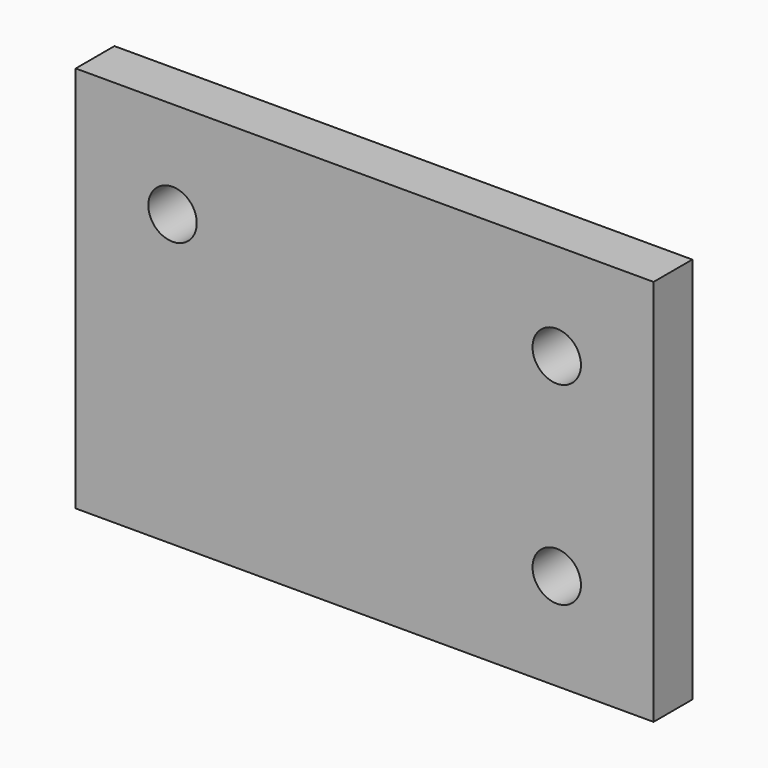
from build123d import *

# Parameters (mm, degrees)
F0_R     = 5
F1_DEPTH = 10


# Not quite as in the source:
# - the program builds the solid bodies; features that only make, move or delete a surface that nothing else refers to are left out


with BuildPart() as f1:
    # F0 (on Front) → F1 (new body)
    with BuildSketch(Plane.XZ):
        Polygon((45.889818927, 55.3569364734), (-73.4539608263, 55.3569364734), (-73.4539608263, 35.3569364734), (-73.4539608263, 5.3569364734), (45.889818927, 5.3569364734), (45.889818927, 35.3569364734), align=None)
        with BuildLine():
            ThreePointArc((-48.4539608263, 35.3569364734), (-53.4539608263, 30.3569364734), (-58.4539608263, 35.3569364734))
            ThreePointArc((-58.4539608263, 35.3569364734), (-53.4539608263, 40.3569364734), (-48.4539608263, 35.3569364734))
        make_face(mode=Mode.SUBTRACT)
        with Locations((25.889818927, 35.3569364734)):
            Circle(F0_R, mode=Mode.SUBTRACT)
        with BuildLine():
            Line((45.889818927, 5.3569364734), (-73.4539608263, 5.3569364734))
            Line((-73.4539608263, 5.3569364734), (-73.4539608263, -4.6430635266))
            Line((-73.4539608263, -4.6430635266), (20.889818927, -4.6430635266))
            ThreePointArc((20.889818927, -4.6430635266), (25.889818927, 0.3569364734), (30.889818927, -4.6430635266))
            Line((30.889818927, -4.6430635266), (45.889818927, -4.6430635266))
            Line((45.889818927, -4.6430635266), (45.889818927, 5.3569364734))
        make_face()
        with BuildLine():
            Line((20.889818927, -4.6430635266), (-73.4539608263, -4.6430635266))
            Line((-73.4539608263, -4.6430635266), (-73.4539608263, -24.6430635266))
            Line((-73.4539608263, -24.6430635266), (25.4732109606, -24.6430635266))
            Line((25.4732109606, -24.6430635266), (45.889818927, -24.6430635266))
            Line((45.889818927, -24.6430635266), (45.889818927, -4.6430635266))
            Line((45.889818927, -4.6430635266), (30.889818927, -4.6430635266))
            ThreePointArc((30.889818927, -4.6430635266), (25.889818927, -9.6430635266), (20.889818927, -4.6430635266))
        make_face()
    extrude(amount=F1_DEPTH)


solid = f1.part
